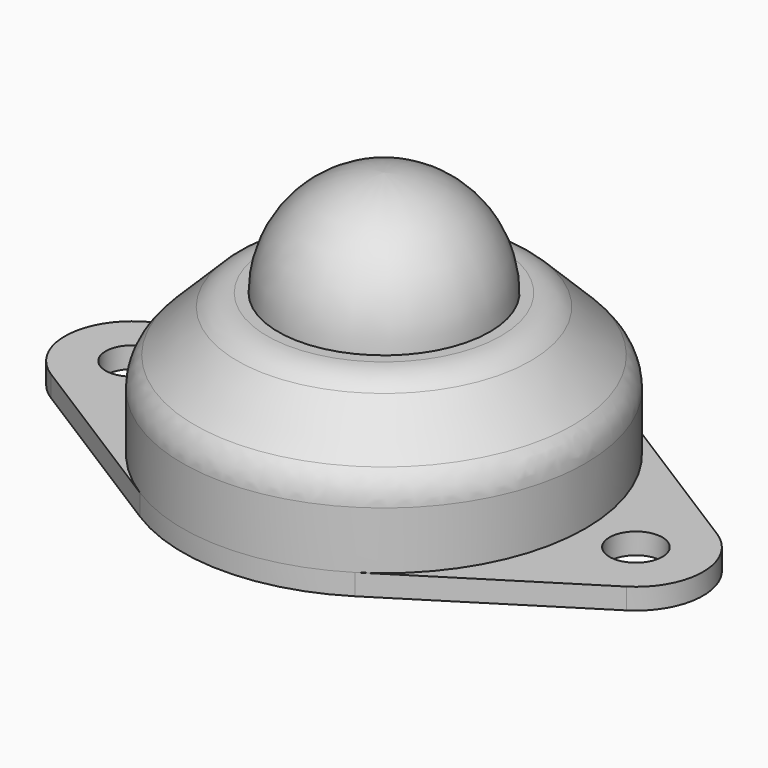
from build123d import *

# Parameters (mm, degrees)
F0_R     = 2
F1_DEPTH = 1.5875
F2_R     = 15.24
F3_DEPTH = 10.7315
F4_R     = 8.001
F5_DEPTH = 8.001
F6_R     = 8.00099
F7_SIZE  = 5.08
F8_R     = 3.175


# Not quite as in the source:
# - a fillet or chamfer is up to 0.001 mm smaller than in the source, because OpenCascade refuses the exact size


with BuildPart() as f1:
    # F0 (on Top) → F1 (new body)
    with BuildSketch(Plane.XY):
        with BuildLine():
            Line((10.922, 12.8915947811), (-2.7093333333, 4.2971982604))
            ThreePointArc((-2.7093333333, 4.2971982604), (-5.08, 0), (-2.7093333333, -4.2971982604))
            Line((-2.7093333333, -4.2971982604), (10.922, -12.8915947811))
            ThreePointArc((10.922, -12.8915947811), (19.05, -15.24), (27.178, -12.8915947811))
            Line((27.178, -12.8915947811), (40.8093333333, -4.2971982604))
            ThreePointArc((40.8093333333, -4.2971982604), (43.18, 0), (40.8093333333, 4.2971982604))
            Line((40.8093333333, 4.2971982604), (27.178, 12.8915947811))
            ThreePointArc((27.178, 12.8915947811), (19.05, 15.24), (10.922, 12.8915947811))
        make_face()
        Circle(F0_R, mode=Mode.SUBTRACT)
        with Locations((38.1, 0)):
            Circle(F0_R, mode=Mode.SUBTRACT)
    extrude(amount=F1_DEPTH)

    # F2 (on face) → F3 (join)
    with BuildSketch(Plane.XY.offset(1.5875)):
        with Locations((19.05, 0)):
            Circle(F2_R)
    extrude(amount=F3_DEPTH)

    # F4 (on face) → F5 (join)
    with BuildSketch(Plane.XY.offset(12.319)):
        with Locations((19.05, 0)):
            Circle(F4_R)
    extrude(amount=F5_DEPTH)

    # F6 (radius 8.001 in the source; OpenCascade refuses exactly that, so slightly less here)
    f6_edges = [f1.edges().sort_by_distance(p)[0] for p in [
        (11.049, 0, 20.32),
    ]]
    fillet(f6_edges, radius=F6_R)

    # F7
    f7_edges = [f1.edges().sort_by_distance(p)[0] for p in [
        (3.81, 0, 12.319),
    ]]
    chamfer(f7_edges, length=F7_SIZE)

    # F8
    f8_edges = [f1.edges().sort_by_distance(p)[0] for p in [
        (3.81, 0, 7.239),
        (8.89, 0, 12.319),
    ]]
    fillet(f8_edges, radius=F8_R)


solid = f1.part
